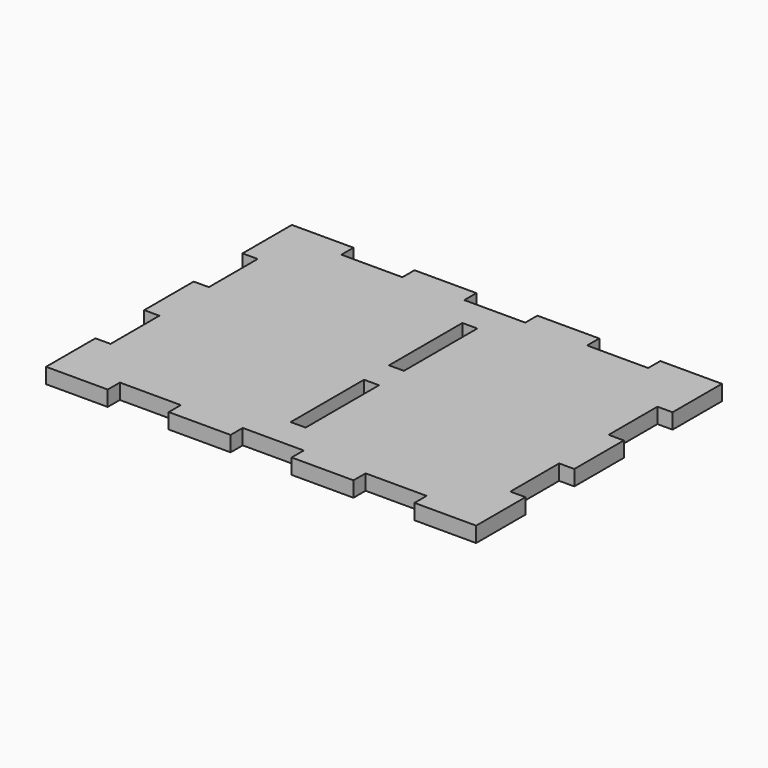
from build123d import *

# Parameters (mm, degrees)
F1_DEPTH = 6.35
F2_W     = 6.1722
F2_H     = 37.9222
F3_DEPTH = 6.351


# Not quite as in the source:
# - a length typed as a fraction of an inch, garbled in the dataset ("3 / 203.2 mm" for 3/8 in), is restored


with BuildPart() as f1:
    # F0 (on Top) → F1 (new body)
    with BuildSketch(Plane.XY):
        Polygon((0, 25.4889), (0, 0), (25.4889, 0), (25.4889, 6.2611), (50.7111, 6.2611), (50.7111, 0), (76.2889, 0), (76.2889, 6.2611), (101.5111, 6.2611), (101.5111, 0), (127.0889, 0), (127.0889, 6.2611), (152.3111, 6.2611), (152.3111, 0), (177.8, 0), (177.8, 25.4889), (171.5389, 25.4889), (171.5389, 50.7111), (177.8, 50.7111), (177.8, 76.2889), (171.5389, 76.2889), (171.5389, 101.5111), (177.8, 101.5111), (177.8, 127), (152.3111, 127), (152.3111, 120.7389), (127.0889, 120.7389), (127.0889, 127), (101.5111, 127), (101.5111, 120.7389), (76.2889, 120.7389), (76.2889, 127), (50.7111, 127), (50.7111, 120.7389), (25.4889, 120.7389), (25.4889, 127), (0, 127), (0, 101.5111), (6.2611, 101.5111), (6.2611, 76.2889), (0, 76.2889), (0, 50.7111), (6.2611, 50.7111), (6.2611, 25.4889), align=None)
    extrude(amount=F1_DEPTH)

    # F2 (on face) → F3 (cut, through all)
    with BuildSketch(Plane.XY.offset(6.35)):
        with Locations((88.9, 88.9)):
            Rectangle(F2_W, F2_H)
        with Locations((88.9, 38.1)):
            Rectangle(F2_W, F2_H)
    extrude(amount=-F3_DEPTH, mode=Mode.SUBTRACT)


solid = f1.part
